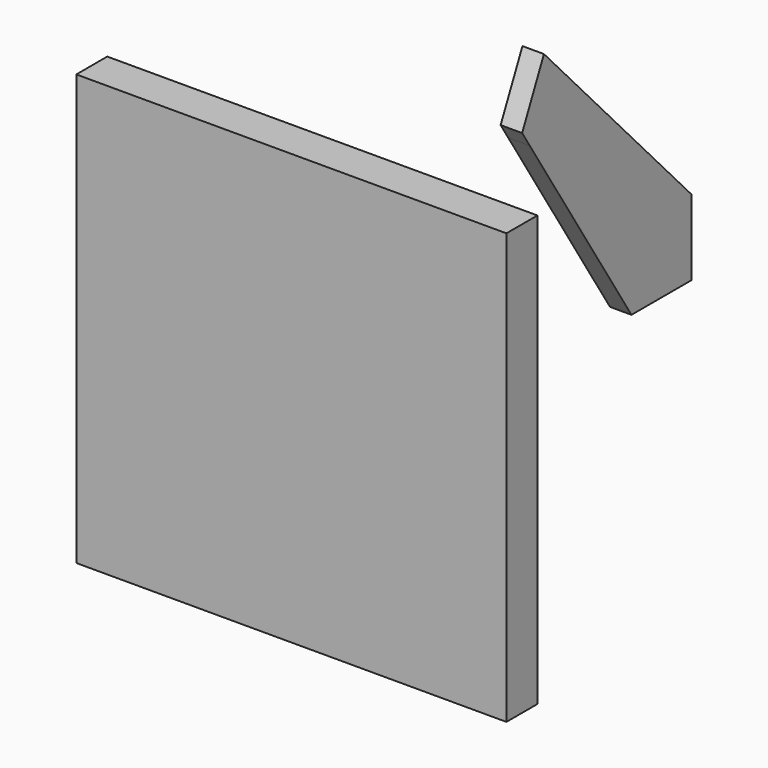
from build123d import *

# Parameters (mm, degrees)
F0_W     = 200
F0_H     = 200
F0_R     = 7.6
F0_W_2   = 128
F0_H_2   = 128
F1_DEPTH = 18
F2_DEPTH = 10
F3_DEPTH = 13.2
F5_START = 45.5
F5_DEPTH = 10


# Not quite as in the source:
# - a feature names something its author has since deleted; it is built from what else it names


with BuildPart() as f1:
    # F0 (on Front) → F1 (new body)
    with BuildSketch(Plane.XZ):
        Rectangle(F0_W, F0_H)
        with Locations((-76, -76)):
            Circle(F0_R, mode=Mode.SUBTRACT)
        with Locations((-38, -76)):
            Circle(F0_R, mode=Mode.SUBTRACT)
        with Locations((-76, -38)):
            Circle(F0_R, mode=Mode.SUBTRACT)
        with Locations((0, -76)):
            Circle(F0_R, mode=Mode.SUBTRACT)
        with Locations((38, -76)):
            Circle(F0_R, mode=Mode.SUBTRACT)
        with Locations((76, -76)):
            Circle(F0_R, mode=Mode.SUBTRACT)
        with Locations((76, -38)):
            Circle(F0_R, mode=Mode.SUBTRACT)
        with Locations((-76, 0)):
            Circle(F0_R, mode=Mode.SUBTRACT)
        with Locations((-76, 38)):
            Circle(F0_R, mode=Mode.SUBTRACT)
        with Locations((-76, 76)):
            Circle(F0_R, mode=Mode.SUBTRACT)
        with Locations((-38, 76)):
            Circle(F0_R, mode=Mode.SUBTRACT)
        Rectangle(F0_W_2, F0_H_2, mode=Mode.SUBTRACT)
        with Locations((76, 0)):
            Circle(F0_R, mode=Mode.SUBTRACT)
        with Locations((76, 38)):
            Circle(F0_R, mode=Mode.SUBTRACT)
        with Locations((0, 76)):
            Circle(F0_R, mode=Mode.SUBTRACT)
        with Locations((38, 76)):
            Circle(F0_R, mode=Mode.SUBTRACT)
        with Locations((76, 76)):
            Circle(F0_R, mode=Mode.SUBTRACT)
        Rectangle(F0_W_2, F0_H_2)
        with Locations((-38, -38)):
            Circle(F0_R, mode=Mode.SUBTRACT)
        with Locations((0, -38)):
            Circle(F0_R, mode=Mode.SUBTRACT)
        with Locations((38, -38)):
            Circle(F0_R, mode=Mode.SUBTRACT)
        with Locations((-38, 0)):
            Circle(F0_R, mode=Mode.SUBTRACT)
        with Locations((-38, 38)):
            Circle(F0_R, mode=Mode.SUBTRACT)
        Circle(F0_R, mode=Mode.SUBTRACT)
        with Locations((38, 0)):
            Circle(F0_R, mode=Mode.SUBTRACT)
        with Locations((0, 38)):
            Circle(F0_R, mode=Mode.SUBTRACT)
        with Locations((38, 38)):
            Circle(F0_R, mode=Mode.SUBTRACT)
        with Locations((-76, 76)):
            Circle(F0_R)
        with Locations((-76, 38)):
            Circle(F0_R)
        with Locations((-76, 0)):
            Circle(F0_R)
        with Locations((-76, -38)):
            Circle(F0_R)
        with Locations((-76, -76)):
            Circle(F0_R)
        with Locations((-38, -76)):
            Circle(F0_R)
        with Locations((-38, -38)):
            Circle(F0_R)
        with Locations((-38, 0)):
            Circle(F0_R)
        Circle(F0_R)
        with Locations((0, 38)):
            Circle(F0_R)
        with Locations((0, 76)):
            Circle(F0_R)
        with Locations((38, 76)):
            Circle(F0_R)
        with Locations((38, 38)):
            Circle(F0_R)
        with Locations((38, 0)):
            Circle(F0_R)
        with Locations((38, -38)):
            Circle(F0_R)
        with Locations((38, -76)):
            Circle(F0_R)
        with Locations((76, -76)):
            Circle(F0_R)
        with Locations((76, -38)):
            Circle(F0_R)
        with Locations((76, 38)):
            Circle(F0_R)
        with Locations((76, 76)):
            Circle(F0_R)
        with Locations((-38, 76)):
            Circle(F0_R)
        with Locations((0, -38)):
            Circle(F0_R)
        with Locations((0, -76)):
            Circle(F0_R)
        with Locations((76, 0)):
            Circle(F0_R)
        with Locations((-38, 38)):
            Circle(F0_R)
    extrude(amount=F1_DEPTH)

    # F0 (on Front) → F2 (cut)
    with BuildSketch(Plane.XZ):
        Rectangle(F0_W_2, F0_H_2)
        with Locations((-38, -38)):
            Circle(F0_R, mode=Mode.SUBTRACT)
        with Locations((0, -38)):
            Circle(F0_R, mode=Mode.SUBTRACT)
        with Locations((38, -38)):
            Circle(F0_R, mode=Mode.SUBTRACT)
        with Locations((-38, 0)):
            Circle(F0_R, mode=Mode.SUBTRACT)
        with Locations((-38, 38)):
            Circle(F0_R, mode=Mode.SUBTRACT)
        Circle(F0_R, mode=Mode.SUBTRACT)
        with Locations((38, 0)):
            Circle(F0_R, mode=Mode.SUBTRACT)
        with Locations((0, 38)):
            Circle(F0_R, mode=Mode.SUBTRACT)
        with Locations((38, 38)):
            Circle(F0_R, mode=Mode.SUBTRACT)
    extrude(amount=F2_DEPTH, mode=Mode.SUBTRACT)

    # F0 (on Front) → F3 (cut)
    with BuildSketch(Plane.XZ):
        with Locations((76, 76)):
            Circle(F0_R)
        with Locations((38, 76)):
            Circle(F0_R)
        with Locations((38, 38)):
            Circle(F0_R)
        with Locations((76, 38)):
            Circle(F0_R)
        with Locations((76, 0)):
            Circle(F0_R)
        with Locations((76, -38)):
            Circle(F0_R)
        with Locations((38, -38)):
            Circle(F0_R)
        with Locations((38, 0)):
            Circle(F0_R)
        with Locations((76, -76)):
            Circle(F0_R)
        with Locations((38, -76)):
            Circle(F0_R)
        with Locations((0, -76)):
            Circle(F0_R)
        with Locations((0, -38)):
            Circle(F0_R)
        Circle(F0_R)
        with Locations((0, 38)):
            Circle(F0_R)
        with Locations((-38, 76)):
            Circle(F0_R)
        with Locations((0, 76)):
            Circle(F0_R)
        with Locations((-38, 38)):
            Circle(F0_R)
        with Locations((-38, 0)):
            Circle(F0_R)
        with Locations((-38, -38)):
            Circle(F0_R)
        with Locations((-38, -76)):
            Circle(F0_R)
        with Locations((-76, -76)):
            Circle(F0_R)
        with Locations((-76, -38)):
            Circle(F0_R)
        with Locations((-76, 0)):
            Circle(F0_R)
        with Locations((-76, 38)):
            Circle(F0_R)
        with Locations((-76, 76)):
            Circle(F0_R)
    extrude(amount=F3_DEPTH, mode=Mode.SUBTRACT)


with BuildPart() as f5:
    # F4 (on Right) → F5 (new body)
    with BuildSketch(Plane.YZ.offset(F5_START)):
        Polygon((59.4276164012, 127.4429346418), (46.749068549, 100.2537010307), (51.1992318351, 93.233695913), (110.3024893999, 0), (145.3024893999, 0), (145.3024893999, 35), (64.5699502421, 121.907294069), align=None)
    extrude(amount=F5_DEPTH)


solid = Compound([f1.part, f5.part])
